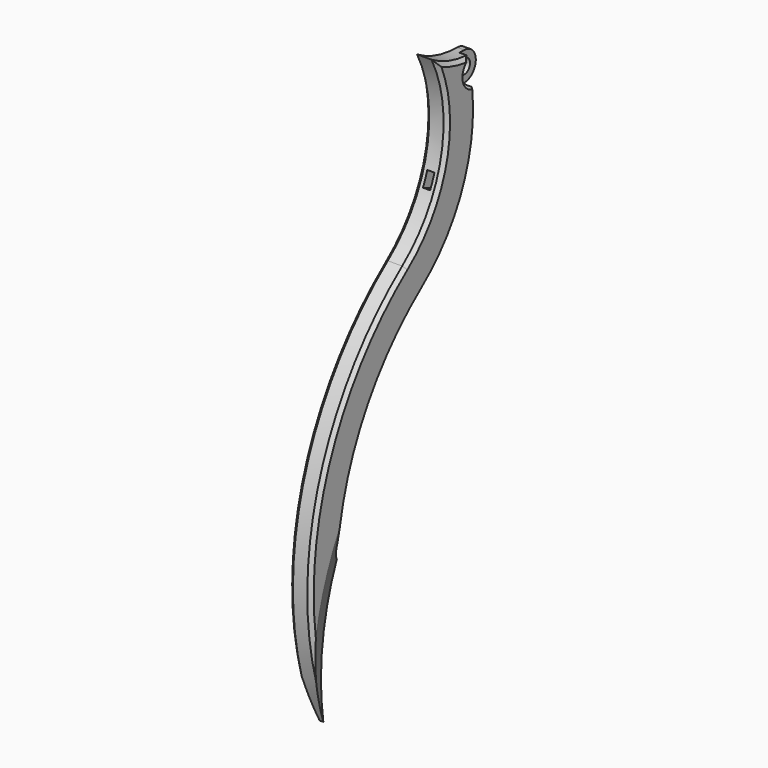
from build123d import *

# Parameters (mm, degrees)
F1_DEPTH    = 3
F2_SIZE     = 0.5
F3_R        = 2.2
F4_DEPTH    = 1.5
F5_R        = 1
F6_DEPTH    = 25
F7_T2_ANGLE = 66.979105944
F7_T4_ANGLE = 66.979105944
F9_START    = -1
F9_DEPTH    = 1


# Not quite as in the source:
# - a fillet or chamfer that OpenCascade refuses, or shapes differently, is made with other operations: its cross-section is extruded or revolved along the edge and cut away or added


with BuildPart() as f1:
    # F0 (on Right) → F1 (new body)
    with BuildSketch(Plane.YZ):
        with BuildLine():
            ThreePointArc((0, -2), (1.4142135624, -1.4142135624), (2, 0))
            ThreePointArc((2, 0), (1.4142135624, 1.4142135624), (0, 2))
            ThreePointArc((0, 2), (-2, 0), (0, -2))
        make_face()
        with BuildLine():
            ThreePointArc((0, -2), (-2, 0), (0, 2))
            ThreePointArc((0, 2), (-3.6215795528, 2.5039519212), (-6.9679827429, 3.9775162004))
            ThreePointArc((-6.9679827429, 3.9775162004), (-5.2841991645, -8.562454479), (-12.0608618515, -19.247155439))
            ThreePointArc((-12.0608618515, -19.247155439), (-27.2940486142, -42.4780574149), (-24.8540620048, -70.1506295922))
            ThreePointArc((-24.8540620048, -70.1506295922), (-24.9977932498, -60.4898051339), (-22.5043967366, -51.1551834643))
            ThreePointArc((-22.5043967366, -51.1551834643), (-23.2047477115, -50.1129852075), (-23.3636565752, -48.8674264303))
            ThreePointArc((-23.3636565752, -48.8674264303), (-18.817838904, -34.5662944148), (-9.0101721364, -23.2086314596))
            ThreePointArc((-9.0101721364, -23.2086314596), (-1.7247742588, -13.7854899156), (0, -2))
        make_face()
    extrude(amount=F1_DEPTH)

    # F2
    f2_edges = [f1.edges().sort_by_distance(p)[0] for p in [
        (3, 2, 0),
        (3, -3.62158, 2.503952),
        (3, -5.284199, -8.562454),
        (3, -27.294049, -42.478057),
        (3, -24.997793, -60.489805),
        (3, -23.204748, -50.112985),
        (3, -18.817839, -34.566294),
        (3, -1.724774, -13.78549),
        (0, 2, 0),
        (0, -3.62158, 2.503952),
        (0, -5.284199, -8.562454),
        (0, -27.294049, -42.478057),
        (0, -24.997793, -60.489805),
        (0, -23.204748, -50.112985),
        (0, -18.817839, -34.566294),
        (0, -1.724774, -13.78549),
    ]]
    chamfer(f2_edges, length=F2_SIZE)

    # F3 (on face) → F4 (cut)
    with BuildSketch(Plane.YZ.offset(3)):
        Circle(F3_R)
    extrude(amount=-F4_DEPTH, mode=Mode.SUBTRACT)

    # F5 (on face) → F6 (cut)
    with BuildSketch(Plane.YZ.offset(1.5)):
        Circle(F5_R)
    extrude(amount=-F6_DEPTH, mode=Mode.SUBTRACT)

    # F7: chamfer of 2.5 on 2 edges, made by hand

    # F7_s1 → F7_t2 (revolve, cut)
    with BuildSketch(Plane(origin=(0, 33.2597277938, -48.8887943232), x_dir=(1, 0, 0), z_dir=(0, 0.5624874969, -0.8268057909))):
        Polygon((0, 66.4232158642), (1.767766953, 62.1554489112), (0, 63.9232158642), align=None)
    revolve(axis=Axis((0, 9.8679252657, -64.8025634284), (-1, 0, 0)), revolution_arc=F7_T2_ANGLE, mode=Mode.SUBTRACT)

    # F7_s3 → F7_t4 (revolve, cut)
    with BuildSketch(Plane(origin=(0, 33.2597277938, -48.8887943232), x_dir=(1, 0, 0), z_dir=(0, 0.5624874969, -0.8268057909))):
        Polygon((3, 66.4232158642), (1.232233047, 62.1554489112), (3, 63.9232158642), align=None)
    revolve(axis=Axis((3, 9.8679252657, -64.8025634284), (-1, 0, 0)), revolution_arc=F7_T4_ANGLE, mode=Mode.SUBTRACT)

    # F8 (on face) → F9 (cut)
    with BuildSketch(Plane.YZ.offset(3).offset(F9_START)):
        with BuildLine():
            ThreePointArc((14, 0), (0, 14), (-14, 0))
            ThreePointArc((-14, 0), (0, -14), (14, 0))
        make_face()
        with BuildLine():
            ThreePointArc((-12, 0), (0, 12), (12, 0))
            ThreePointArc((12, 0), (0, -12), (-12, 0))
        make_face(mode=Mode.SUBTRACT)
    extrude(amount=-F9_DEPTH, mode=Mode.SUBTRACT)


solid = f1.part
